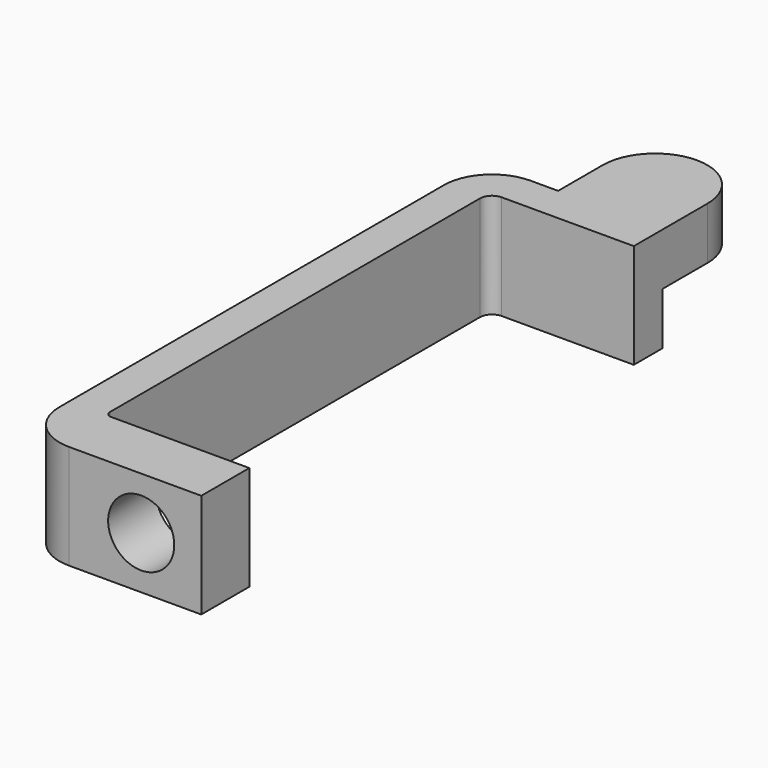
from build123d import *

# Parameters (mm, degrees)
F0_W     = 24
F0_H     = 6
F0_H_2   = 10
F1_DEPTH = 17.4
F2_R     = 8
F3_R     = 2
F5_R     = 5.5
F6_DEPTH = 25
F7_R     = 1
F4_W     = 17.4
F4_H     = 8.7
F8_DEPTH = 18
F9_R     = 8.69999


# Not quite as in the source:
# - a fillet or chamfer is up to 0.001 mm smaller than in the source, because OpenCascade refuses the exact size


with BuildPart() as f1:
    # F0 (on Top) → F1 (new body)
    with BuildSketch(Plane.XY):
        Polygon((3, 41.0029157541), (3, 47.0029157541), (-3, 47.0029157541), (-3, -48.9970842459), (3, -48.9970842459), (3, -38.9970842459), align=None)
        with Locations((15, 44.0029157541)):
            Rectangle(F0_W, F0_H)
        with Locations((15, -43.9970842459)):
            Rectangle(F0_W, F0_H_2)
    extrude(amount=F1_DEPTH)

    # F2
    f2_edges = [f1.edges().sort_by_distance(p)[0] for p in [
        (-3, 47.002916, 8.7),
        (-3, -48.997084, 8.7),
    ]]
    fillet(f2_edges, radius=F2_R)

    # F3
    f3_edges = [f1.edges().sort_by_distance(p)[0] for p in [
        (3, 41.002916, 8.7),
    ]]
    fillet(f3_edges, radius=F3_R)

    # F5 (on face) → F6 (cut)
    with BuildSketch(Plane.XZ.offset(48.9970842459)):
        with Locations((17, 8.7)):
            Circle(F5_R)
    extrude(amount=-F6_DEPTH, mode=Mode.SUBTRACT)

    # F7
    f7_edges = [f1.edges().sort_by_distance(p)[0] for p in [
        (3, -38.997084, 8.7),
    ]]
    fillet(f7_edges, radius=F7_R)

    # F4 (on face) → F8 (join)
    with BuildSketch(Plane(origin=(0, 47.0029157541, 0), x_dir=(-1, 0, 0), z_dir=(0, 1, 0))):
        with Locations((-18.3, 13.05)):
            Rectangle(F4_W, F4_H)
    extrude(amount=F8_DEPTH)

    # F9 (radius 8.7 in the source; OpenCascade refuses exactly that, so slightly less here)
    f9_edges = [f1.edges().sort_by_distance(p)[0] for p in [
        (27, 65.002916, 13.05),
        (9.6, 65.002916, 13.05),
    ]]
    fillet(f9_edges, radius=F9_R)


solid = f1.part
